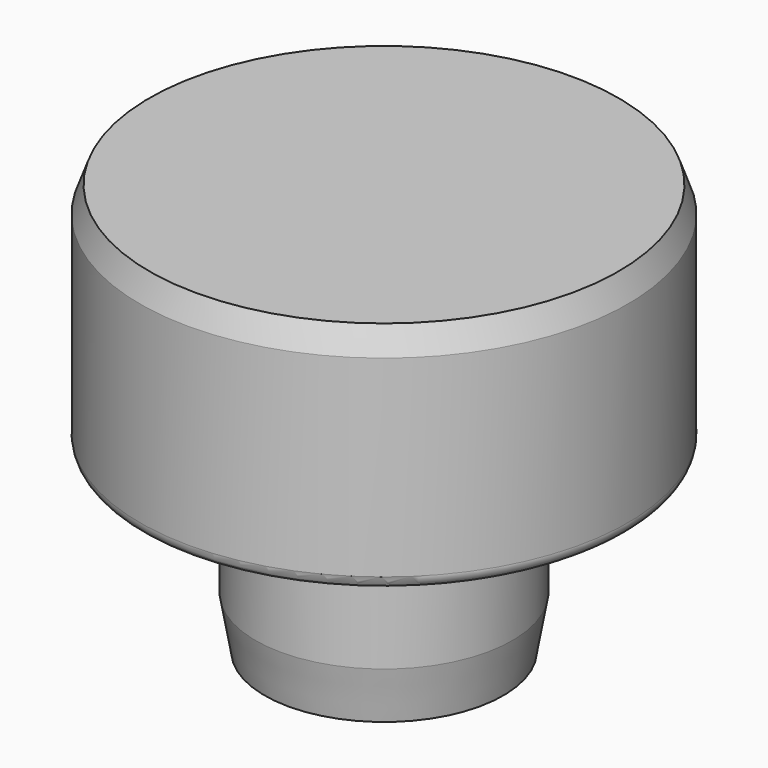
from build123d import *

# Parameters (mm, degrees)
F3_R     = 0.25
F4_SIZE2 = 0.1763269807
F4_SIZE  = 1
F6_D     = 3
F6_DEPTH = 3
F6_TIP   = 0.9012909285


# Not quite as in the source:
# - a fillet or chamfer that OpenCascade refuses, or shapes differently, is made with other operations: its cross-section is extruded or revolved along the edge and cut away or added


with BuildPart() as f1:
    # F0 (on Right) → F1 (revolve)
    with BuildSketch(Plane.YZ):
        Polygon((0, 0), (-4.75, 0), (-4.75, -4.5), (-2.5, -4.5), (-2.5, -8), (0, -8), align=None)
    revolve(axis=Axis((0, 0, -4), (0, 0, -1)))

    # F2: chamfer of 0.5 x 0.1819851171 on 1 edges, made by hand

    # F2_s1 → F2_t2 (revolve, cut)
    with BuildSketch(Plane.YZ):
        Polygon((-4.5680148829, 0), (-4.75, -0.5), (-4.75, 0), align=None)
    revolve(axis=Axis((0, 0, 0), (0, 0, -1)), mode=Mode.SUBTRACT)

    # F3
    f3_edges = [f1.edges().sort_by_distance(p)[0] for p in [
        (0, 4.75, -4.5),
        (0, 2.5, -4.5),
    ]]
    fillet(f3_edges, radius=F3_R)

    # F4
    f4_edges = [f1.edges().sort_by_distance(p)[0] for p in [
        (0, 2.5, -8),
    ]]
    chamfer(f4_edges, length=F4_SIZE, length2=F4_SIZE2)

    # F6
    with Locations(Plane(origin=(0, 0, -8), x_dir=(1, 0, 0), z_dir=(0, 0, -1))):
        with Locations((0, 0)):
            Hole(F6_D / 2, depth=F6_DEPTH)
            with Locations((0, 0, -(F6_DEPTH + F6_TIP / 2))):  # 118° drill point
                Cone(0, F6_D / 2, F6_TIP, mode=Mode.SUBTRACT)


solid = f1.part
